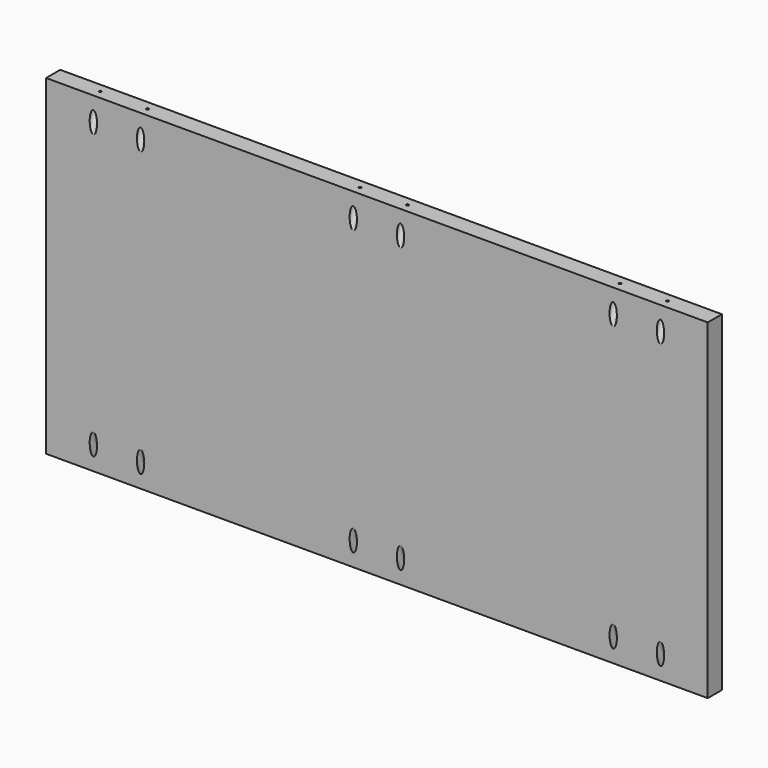
from build123d import *

# Parameters (mm, degrees)
F0_W     = 711.2
F0_H     = 355.6
F1_DEPTH = 19.05
F5_DEPTH = 25.4
F7_D     = 2.54


# Not quite as in the source:
# - a pattern or mirror of a feature is missing from the dataset's text; its kind, count and spacing are read off the source's solid


with BuildPart() as f1:
    # F0 (on Front) → F1 (new body)
    with BuildSketch(Plane.XZ):
        with Locations((355.6, 177.8)):
            Rectangle(F0_W, F0_H)
    extrude(amount=F1_DEPTH)

    # F4 (on face) → F5 (cut, symmetric)
    with BuildSketch(Plane(origin=(0, 103.89580768, 285.4513855767), x_dir=(1, 0, 0), z_dir=(0, 0.3420201433, 0.9396926208))):
        with BuildLine():
            ThreePointArc((664.337, -130.8361957521), (660.4, -126.8991957521), (656.463, -130.8361957521))
            Line((656.463, -130.8361957521), (664.337, -130.8361957521))
        make_face()
        with BuildLine():
            Line((664.337, -130.8361957521), (656.463, -130.8361957521))
            ThreePointArc((656.463, -130.8361957521), (660.4, -134.7731957521), (664.337, -130.8361957521))
        make_face()
        with BuildLine():
            ThreePointArc((613.537, -130.8361957521), (609.6, -126.8991957521), (605.663, -130.8361957521))
            Line((605.663, -130.8361957521), (613.537, -130.8361957521))
        make_face()
        with BuildLine():
            Line((613.537, -130.8361957521), (605.663, -130.8361957521))
            ThreePointArc((605.663, -130.8361957521), (609.6, -134.7731957521), (613.537, -130.8361957521))
        make_face()
        with BuildLine():
            ThreePointArc((384.937, -130.8361957521), (381, -126.8991957521), (377.063, -130.8361957521))
            Line((377.063, -130.8361957521), (384.937, -130.8361957521))
        make_face()
        with BuildLine():
            Line((384.937, -130.8361957521), (377.063, -130.8361957521))
            ThreePointArc((377.063, -130.8361957521), (381, -134.7731957521), (384.937, -130.8361957521))
        make_face()
        with BuildLine():
            ThreePointArc((326.263, -130.8361957521), (330.2, -134.7731957521), (334.137, -130.8361957521))
            Line((334.137, -130.8361957521), (326.263, -130.8361957521))
        make_face()
        with BuildLine():
            Line((326.263, -130.8361957521), (334.137, -130.8361957521))
            ThreePointArc((334.137, -130.8361957521), (330.2, -126.8991957521), (326.263, -130.8361957521))
        make_face()
        with BuildLine():
            ThreePointArc((46.863, -130.8361957521), (50.8, -134.7731957521), (54.737, -130.8361957521))
            Line((54.737, -130.8361957521), (46.863, -130.8361957521))
        make_face()
        with BuildLine():
            Line((46.863, -130.8361957521), (54.737, -130.8361957521))
            ThreePointArc((54.737, -130.8361957521), (50.8, -126.8991957521), (46.863, -130.8361957521))
        make_face()
        with BuildLine():
            ThreePointArc((97.663, -130.8361957521), (101.6, -134.7731957521), (105.537, -130.8361957521))
            Line((105.537, -130.8361957521), (97.663, -130.8361957521))
        make_face()
        with BuildLine():
            Line((97.663, -130.8361957521), (105.537, -130.8361957521))
            ThreePointArc((105.537, -130.8361957521), (101.6, -126.8991957521), (97.663, -130.8361957521))
        make_face()
    f5 = extrude(amount=F5_DEPTH, both=True, mode=Mode.SUBTRACT)

    # F5_copies: F5 across plane
    add(f5.mirror(Plane(origin=(1e-06, 1.5e-05, 177.800048), x_dir=(-1, 0, 0), z_dir=(0, 0, -1))), mode=Mode.SUBTRACT)

    # F7 (through all)
    with Locations(Plane(origin=(0, 112.5831193204, 309.3195781446), x_dir=(1, 0, 0), z_dir=(0, -0.3420201433, -0.9396926208))):
        with Locations((660.4, 130.8361957521), (609.6, 130.8361957521), (381, 130.8361957521), (330.2, 130.8361957521), (101.6, 130.8361957521), (50.8, 130.8361957521)):
            f7 = Hole(F7_D / 2)

    # F7_copies: F7 across plane
    add(f7.mirror(Plane(origin=(0, -1e-06, 177.800002), x_dir=(-1, 0, 0), z_dir=(0, 0, -1))), mode=Mode.SUBTRACT)


solid = f1.part
